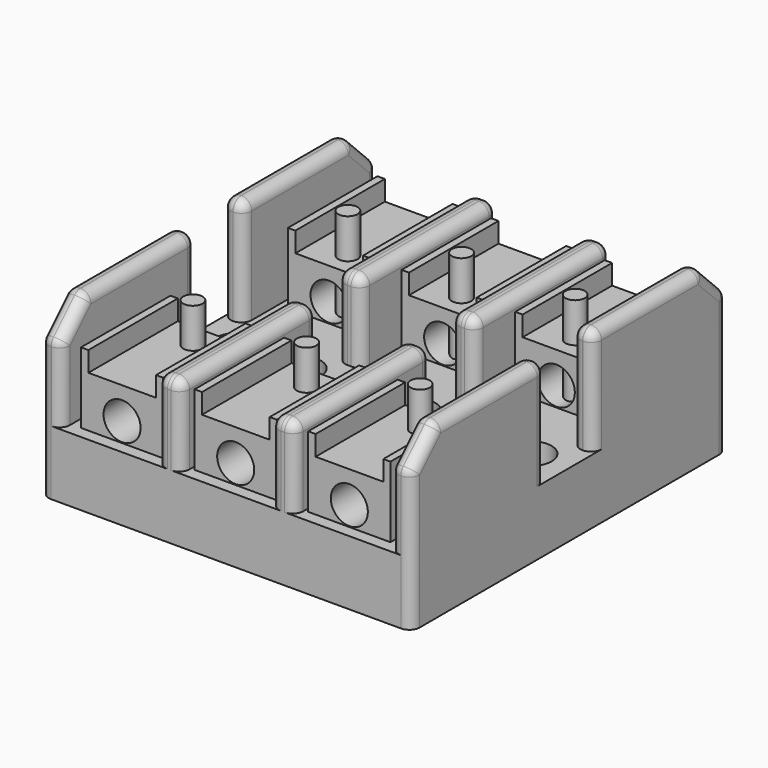
from build123d import *

# Parameters (mm, degrees)
F0_W      = 115
F0_H      = 122.5
F1_DEPTH  = 20
F2_R      = 6.5
F3_DEPTH  = 18
F4_R      = 2.8
F5_DEPTH  = 20.001
F6_W      = 25.5
F6_H      = 34.7
F7_DEPTH  = 22
F8_W      = 6.5
F8_H      = 52
F9_DEPTH  = 33
F10_W     = 7.5
F10_H     = 52.7
F11_DEPTH = 25
F12_R     = 3
F13_DEPTH = 28.1
F14_R     = 5.75
F15_DEPTH = 122.501
F16_W     = 21
F16_H     = 34.7
F17_DEPTH = 6.2
F18_W     = 21
F18_H     = 34.7
F19_DEPTH = 6.2
F20_W     = 21
F20_H     = 34.7
F21_DEPTH = 6.2
F22_W     = 21
F22_H     = 34.7
F23_DEPTH = 6.2
F24_W     = 21
F24_H     = 34.7
F25_DEPTH = 6.2
F26_W     = 21
F26_H     = 34.7
F27_DEPTH = 6.2
F28_SIZE  = 10
F29_R     = 3.2


with BuildPart() as f1:
    # F0 (on Top) → F1 (new body)
    with BuildSketch(Plane.XY):
        with Locations((57.5, 61.25)):
            Rectangle(F0_W, F0_H)
    extrude(amount=F1_DEPTH)

    # F2 (on face) → F3 (cut)
    with BuildSketch(Plane.XY.offset(20)):
        with Locations((12, 61.25)):
            Circle(F2_R)
        with Locations((31.4, 61.25)):
            Circle(F2_R)
        with Locations((48.1, 61.25)):
            Circle(F2_R)
        with Locations((103, 61.25)):
            Circle(F2_R)
        with Locations((83.6, 61.25)):
            Circle(F2_R)
        with Locations((66.9, 61.25)):
            Circle(F2_R)
    extrude(amount=-F3_DEPTH, mode=Mode.SUBTRACT)

    # F4 (on face) → F5 (cut, through all)
    with BuildSketch(Plane.XY.offset(20)):
        with Locations((12, 61.25)):
            Circle(F4_R)
        with Locations((31.4, 61.25)):
            Circle(F4_R)
        with Locations((48.1, 61.25)):
            Circle(F4_R)
        with Locations((66.9, 61.25)):
            Circle(F4_R)
        with Locations((83.6, 61.25)):
            Circle(F4_R)
        with Locations((103, 61.25)):
            Circle(F4_R)
    extrude(amount=-F5_DEPTH, mode=Mode.SUBTRACT)

    # F6 (on face) → F7 (join)
    with BuildSketch(Plane.XY.offset(20)):
        with Locations((22.25, 101.35)):
            Rectangle(F6_W, F6_H)
        with Locations((57.5, 101.35)):
            Rectangle(F6_W, F6_H)
        with Locations((92.75, 101.35)):
            Rectangle(F6_W, F6_H)
        with Locations((22.25, 21.083796525)):
            Rectangle(F6_W, F6_H)
        with Locations((57.5, 21.083796525)):
            Rectangle(F6_W, F6_H)
        with Locations((92.75, 21.083796525)):
            Rectangle(F6_W, F6_H)
    extrude(amount=F7_DEPTH)

    # F8 (on face) → F9 (join)
    with BuildSketch(Plane.XY.offset(20)):
        with Locations((3.25, 26)):
            Rectangle(F8_W, F8_H)
        with Locations((111.75, 96.5)):
            Rectangle(F8_W, F8_H)
        with Locations((111.75, 26)):
            Rectangle(F8_W, F8_H)
        with Locations((3.25, 96.5)):
            Rectangle(F8_W, F8_H)
    extrude(amount=F9_DEPTH)

    # F10 (on face) → F11 (join)
    with BuildSketch(Plane.XY.offset(20)):
        with Locations((39.88, 96.15)):
            Rectangle(F10_W, F10_H)
        with Locations((39.88, 26.35)):
            Rectangle(F10_W, F10_H)
        with Locations((75.13, 96.15)):
            Rectangle(F10_W, F10_H)
        with Locations((75.13, 26.35)):
            Rectangle(F10_W, F10_H)
    extrude(amount=F11_DEPTH)

    # F14 (on face) → F15 (cut, through all)
    with BuildSketch(Plane.XZ):
        with Locations((22.25, 26)):
            Circle(F14_R)
        with Locations((57.5, 26)):
            Circle(F14_R)
        with Locations((92.75, 26)):
            Circle(F14_R)
    extrude(amount=-F15_DEPTH, mode=Mode.SUBTRACT)

    # F16 (on face) → F17 (cut)
    with BuildSketch(Plane.XY.offset(42)):
        with Locations((22.3, 21.083796525)):
            Rectangle(F16_W, F16_H)
    extrude(amount=-F17_DEPTH, mode=Mode.SUBTRACT)

    # F18 (on face) → F19 (cut)
    with BuildSketch(Plane.XY.offset(42)):
        with Locations((57.55, 21.083796525)):
            Rectangle(F18_W, F18_H)
    extrude(amount=-F19_DEPTH, mode=Mode.SUBTRACT)

    # F20 (on face) → F21 (cut)
    with BuildSketch(Plane.XY.offset(42)):
        with Locations((92.8, 21.083796525)):
            Rectangle(F20_W, F20_H)
    extrude(amount=-F21_DEPTH, mode=Mode.SUBTRACT)

    # F22 (on face) → F23 (cut)
    with BuildSketch(Plane.XY.offset(42)):
        with Locations((22.3, 101.35)):
            Rectangle(F22_W, F22_H)
    extrude(amount=-F23_DEPTH, mode=Mode.SUBTRACT)

    # F24 (on face) → F25 (cut)
    with BuildSketch(Plane.XY.offset(42)):
        with Locations((57.55, 101.35)):
            Rectangle(F24_W, F24_H)
    extrude(amount=-F25_DEPTH, mode=Mode.SUBTRACT)

    # F26 (on face) → F27 (cut)
    with BuildSketch(Plane.XY.offset(42)):
        with Locations((92.8, 101.35)):
            Rectangle(F26_W, F26_H)
    extrude(amount=-F27_DEPTH, mode=Mode.SUBTRACT)

    # F28
    f28_edges = [f1.edges().sort_by_distance(p)[0] for p in [
        (3.25, 0, 53),
        (111.75, 0, 53),
        (111.75, 122.5, 53),
        (3.25, 122.5, 53),
    ]]
    chamfer(f28_edges, length=F28_SIZE)

    # F29
    f29_edges = [f1.edges().sort_by_distance(p)[0] for p in [
        (6.5, 91.5, 53),
        (3.25, 70.5, 53),
        (0, 91.5, 53),
        (39.88, 122.5, 45),
        (36.13, 96.15, 45),
        (39.88, 69.8, 45),
        (43.63, 96.15, 45),
        (75.13, 122.5, 45),
        (71.38, 96.15, 45),
        (75.13, 69.8, 45),
        (78.88, 96.15, 45),
        (75.13, 0, 45),
        (78.88, 26.35, 45),
        (75.13, 52.7, 45),
        (71.38, 26.35, 45),
        (36.13, 26.35, 45),
        (39.88, 0, 45),
        (43.63, 26.35, 45),
        (39.88, 52.7, 45),
        (0, 31, 53),
        (3.25, 10, 53),
        (3.25, 52, 53),
        (6.5, 31, 53),
        (0, 5, 48),
        (3.25, 0, 43),
        (6.5, 5, 48),
        (108.5, 5, 48),
        (111.75, 0, 43),
        (111.75, 10, 53),
        (115, 5, 48),
        (115, 31, 53),
        (111.75, 52, 53),
        (108.5, 31, 53),
        (115, 91.5, 53),
        (111.75, 112.5, 53),
        (111.75, 70.5, 53),
        (108.5, 91.5, 53),
        (78.88, 0, 32.5),
        (71.38, 0, 32.5),
        (43.63, 0, 32.5),
        (36.13, 0, 32.5),
        (6.5, 0, 31.5),
        (0, 0, 21.5),
        (108.5, 0, 31.5),
        (115, 0, 21.5),
        (115, 52, 36.5),
        (108.5, 52, 36.5),
        (78.88, 52.7, 32.5),
        (71.38, 52.7, 32.5),
        (43.63, 52.7, 32.5),
        (36.13, 52.7, 32.5),
        (6.5, 52, 36.5),
        (0, 52, 36.5),
        (115, 122.5, 21.5),
        (115, 117.5, 48),
        (111.75, 122.5, 43),
        (108.5, 117.5, 48),
        (108.5, 122.5, 31.5),
        (78.88, 122.5, 32.5),
        (71.38, 122.5, 32.5),
        (43.63, 122.5, 32.5),
        (36.13, 122.5, 32.5),
        (6.5, 117.5, 48),
        (3.25, 122.5, 43),
        (3.25, 112.5, 53),
        (0, 117.5, 48),
        (0, 122.5, 21.5),
        (6.5, 122.5, 31.5),
        (115, 70.5, 36.5),
        (108.5, 70.5, 36.5),
        (78.88, 69.8, 32.5),
        (71.38, 69.8, 32.5),
        (43.63, 69.8, 32.5),
        (36.13, 69.8, 32.5),
        (6.5, 70.5, 36.5),
        (0, 70.5, 36.5),
    ]]
    fillet(f29_edges, radius=F29_R)


with BuildPart() as f13:
    # F12 (on face) → F13 (new body)
    with BuildSketch(Plane.XY.offset(20)):
        with Locations((22.5, 91)):
            Circle(F12_R)
    extrude(amount=F13_DEPTH)


with BuildPart() as f13b:
    # F12 (on face) → F13, piece 2 (new body)
    with BuildSketch(Plane.XY.offset(20)):
        with Locations((57.75, 91)):
            Circle(F12_R)
    extrude(amount=F13_DEPTH)


with BuildPart() as f13c:
    # F12 (on face) → F13, piece 3 (new body)
    with BuildSketch(Plane.XY.offset(20)):
        with Locations((93, 91)):
            Circle(F12_R)
    extrude(amount=F13_DEPTH)


with BuildPart() as f13d:
    # F12 (on face) → F13, piece 4 (new body)
    with BuildSketch(Plane.XY.offset(20)):
        with Locations((22.5, 30.8929812312)):
            Circle(F12_R)
    extrude(amount=F13_DEPTH)


with BuildPart() as f13e:
    # F12 (on face) → F13, piece 5 (new body)
    with BuildSketch(Plane.XY.offset(20)):
        with Locations((57.75, 30.8929812312)):
            Circle(F12_R)
    extrude(amount=F13_DEPTH)


with BuildPart() as f13f:
    # F12 (on face) → F13, piece 6 (new body)
    with BuildSketch(Plane.XY.offset(20)):
        with Locations((93, 30.8929812312)):
            Circle(F12_R)
    extrude(amount=F13_DEPTH)


solid = Compound([f1.part, f13.part, f13b.part, f13c.part, f13d.part, f13e.part, f13f.part])
